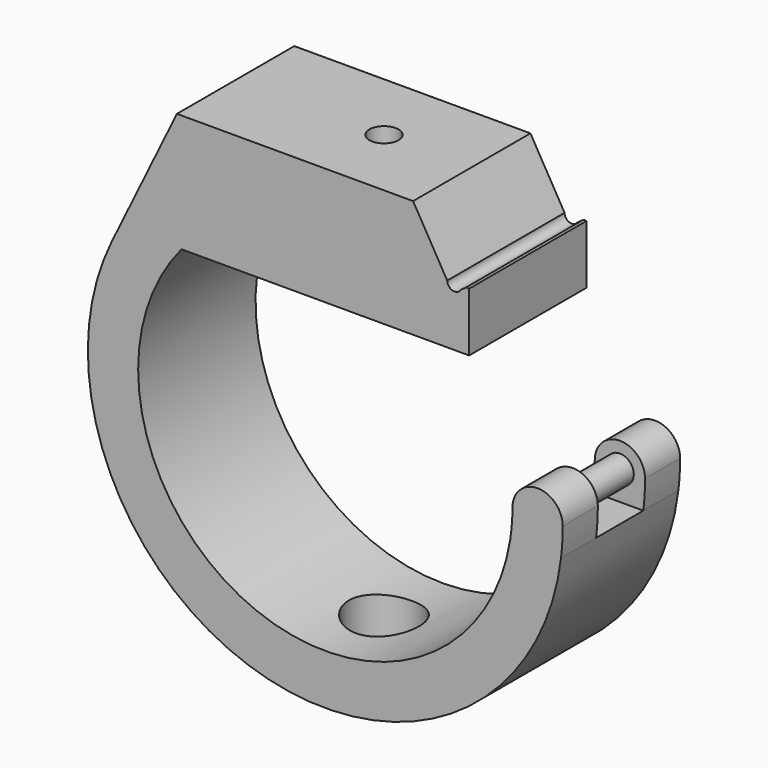
from build123d import *

# Parameters (mm, degrees)
F1_DEPTH  = 7.5
F2_DEPTH  = 17.6
F4_DEPTH  = 7.5
F6_DEPTH  = 25
F7_DEPTH  = 25.1
F8_R      = 2.5
F9_DEPTH  = 121.4
F10_DEPTH = 25.1
F11_R     = 6
F11_R_2   = 2.5
F12_DEPTH = 82
F14_DEPTH = 25.1


# Not quite as in the source:
# - a feature names something its author has since deleted; it is built from what else it names


with BuildPart() as f1:
    # F0 (on Front) → F1 (new body)
    with BuildSketch(Plane.XZ):
        with BuildLine():
            Line((24.609375, 40.625), (-25.390625, 40.625))
            Line((-25.390625, 40.625), (-25.390625, 31.7128804606))
            ThreePointArc((-25.390625, 31.7128804606), (-31.7255791152, 25.3747562511), (-36.5168539326, 17.8019662921))
            ThreePointArc((-36.5168539326, 17.8019662921), (-11.5217513517, -38.9568976022), (40.3254101185, -4.924624227))
            Line((40.3254101185, -4.924624227), (31.6393058234, -4.924624227))
            ThreePointArc((31.6393058234, -4.924624227), (-30.8610352871, -8.5378040369), (24.609375, 20.4860015345))
            Line((24.609375, 20.4860015345), (24.609375, 32.3228910698))
            Line((24.609375, 32.3228910698), (24.609375, 40.625))
        make_face()
        with BuildLine():
            Line((31.6393058234, -4.924624227), (40.3254101185, -4.924624227))
            ThreePointArc((40.3254101185, -4.924624227), (40.5500333604, -2.4668642988), (40.625, 0))
            ThreePointArc((40.625, 0), (36.3226342652, -4.3023657348), (32.0202685305, 0))
            ThreePointArc((32.0202685305, 0), (31.9248857895, -2.469668822), (31.6393058234, -4.924624227))
        make_face()
        with BuildLine():
            Line((38.6976342652, 0), (40.625, 0))
            ThreePointArc((40.625, 0), (36.3226342652, 4.3023657348), (32.0202685305, 0))
            Line((32.0202685305, 0), (33.9476342652, 0))
            ThreePointArc((33.9476342652, 0), (36.3226342652, 2.375), (38.6976342652, 0))
        make_face()
        with BuildLine():
            ThreePointArc((32.0202685305, 0), (36.3226342652, -4.3023657348), (40.625, 0))
            Line((40.625, 0), (38.6976342652, 0))
            ThreePointArc((38.6976342652, 0), (36.3226342652, -2.375), (33.9476342652, 0))
            Line((33.9476342652, 0), (32.0202685305, 0))
        make_face()
    extrude(amount=F1_DEPTH)

    # F0 (on Front) → F2 (join)
    with BuildSketch(Plane.XZ):
        with BuildLine():
            Line((24.609375, 40.625), (-25.390625, 40.625))
            Line((-25.390625, 40.625), (-25.390625, 31.7128804606))
            ThreePointArc((-25.390625, 31.7128804606), (-31.7255791152, 25.3747562511), (-36.5168539326, 17.8019662921))
            ThreePointArc((-36.5168539326, 17.8019662921), (-11.5217513517, -38.9568976022), (40.3254101185, -4.924624227))
            Line((40.3254101185, -4.924624227), (31.6393058234, -4.924624227))
            ThreePointArc((31.6393058234, -4.924624227), (-30.8610352871, -8.5378040369), (24.609375, 20.4860015345))
            Line((24.609375, 20.4860015345), (24.609375, 32.3228910698))
            Line((24.609375, 32.3228910698), (24.609375, 40.625))
        make_face()
    extrude(amount=F2_DEPTH)

    # F3 (on face) → F4 (join)
    with BuildSketch(Plane.XZ.offset(17.6)):
        with BuildLine():
            Line((24.609375, 40.625), (-25.390625, 40.625))
            Line((-25.390625, 40.625), (-25.390625, 31.7128804606))
            ThreePointArc((-25.390625, 31.7128804606), (-19.7822809369, -35.4831225505), (40.3254101185, -4.924624227))
            Line((40.3254101185, -4.924624227), (31.6393058234, -4.924624227))
            ThreePointArc((31.6393058234, -4.924624227), (-30.8610352871, -8.5378040369), (24.609375, 20.4860015345))
            Line((24.609375, 20.4860015345), (24.609375, 32.3228910698))
            Line((24.609375, 32.3228910698), (24.609375, 40.625))
        make_face()
        with BuildLine():
            Line((31.6393058234, -4.924624227), (40.3254101185, -4.924624227))
            ThreePointArc((40.3254101185, -4.924624227), (40.5500333604, -2.4668642988), (40.625, 0))
            ThreePointArc((40.625, 0), (36.3226342652, -4.3023657348), (32.0202685305, 0))
            ThreePointArc((32.0202685305, 0), (31.9248857895, -2.469668822), (31.6393058234, -4.924624227))
        make_face()
        with BuildLine():
            ThreePointArc((32.0202685305, 0), (36.3226342652, -4.3023657348), (40.625, 0))
            Line((40.625, 0), (38.6976342652, 0))
            ThreePointArc((38.6976342652, 0), (36.3226342652, -2.375), (33.9476342652, 0))
            Line((33.9476342652, 0), (32.0202685305, 0))
        make_face()
        with BuildLine():
            Line((38.6976342652, 0), (40.625, 0))
            ThreePointArc((40.625, 0), (36.3226342652, 4.3023657348), (32.0202685305, 0))
            Line((32.0202685305, 0), (33.9476342652, 0))
            ThreePointArc((33.9476342652, 0), (36.3226342652, 2.375), (38.6976342652, 0))
        make_face()
    extrude(amount=F4_DEPTH)

    # F5 (on face) → F6 (join)
    with BuildSketch(Plane.XZ.offset(25.1)):
        with BuildLine():
            Line((-24.609375, 20.4860015345), (24.609375, 20.4860015345))
            ThreePointArc((24.609375, 20.4860015345), (0, 32.0202685305), (-24.609375, 20.4860015345))
        make_face()
    extrude(amount=-F6_DEPTH)

    # F0 (on Front) → F7 (join)
    with BuildSketch(Plane.XZ):
        with BuildLine():
            Line((33.9476342652, 0), (38.6976342652, 0))
            ThreePointArc((38.6976342652, 0), (36.3226342652, 2.375), (33.9476342652, 0))
        make_face()
        with BuildLine():
            ThreePointArc((33.9476342652, 0), (36.3226342652, -2.375), (38.6976342652, 0))
            Line((38.6976342652, 0), (33.9476342652, 0))
        make_face()
    extrude(amount=F7_DEPTH)

    # F8 (on face) → F9 (cut)
    with BuildSketch(Plane.XY.offset(40.625)):
        with Locations((0, -12.55)):
            Circle(F8_R)
    extrude(amount=-F9_DEPTH, mode=Mode.SUBTRACT)

    # F0 (on Front) → F10 (join)
    with BuildSketch(Plane.XZ):
        with BuildLine():
            Line((-25.390625, 31.7128804606), (-25.390625, 40.625))
            Line((-25.390625, 40.625), (-36.5168539326, 17.8019662921))
            ThreePointArc((-36.5168539326, 17.8019662921), (-31.7255791152, 25.3747562511), (-25.390625, 31.7128804606))
        make_face()
    extrude(amount=F10_DEPTH)

    # F11 (on face) → F12 (cut)
    with BuildSketch(Plane(origin=(0, 0, 20.4860015345), x_dir=(1, 0, 0), z_dir=(0, 0, -1))):
        with Locations((0, 12.55)):
            Circle(F11_R)
        with Locations((0, 12.55)):
            Circle(F11_R_2, mode=Mode.SUBTRACT)
    extrude(amount=F12_DEPTH, mode=Mode.SUBTRACT)

    # F13 (on face) → F14 (cut)
    with BuildSketch(Plane.XZ.offset(25.1)):
        with BuildLine():
            ThreePointArc((23.1832968576, 29.9158197188), (23.3145518173, 30.2237646688), (23.359375, 30.5555007673))
            ThreePointArc((23.359375, 30.5555007673), (22.109375, 31.8055007673), (20.859375, 30.5555007673))
            ThreePointArc((20.859375, 30.5555007673), (21.7776389015, 29.35032395), (23.1832968576, 29.9158197188))
        make_face()
        with BuildLine():
            Line((24.085752666, 30.5555007673), (23.359375, 30.5555007673))
            ThreePointArc((23.359375, 30.5555007673), (23.3145518173, 30.2237646688), (23.1832968576, 29.9158197188))
            Line((23.1832968576, 29.9158197188), (24.085752666, 30.5555007673))
        make_face()
        with BuildLine():
            ThreePointArc((20.859375, 30.5555007673), (22.109375, 31.8055007673), (23.359375, 30.5555007673))
            Line((23.359375, 30.5555007673), (24.085752666, 30.5555007673))
            Line((24.085752666, 30.5555007673), (24.609375, 30.5555007673))
            Line((24.609375, 30.5555007673), (24.609375, 40.625))
            Line((24.609375, 40.625), (15.0185888633, 40.625))
            Line((15.0185888633, 40.625), (20.859375, 30.5555007673))
        make_face()
    extrude(amount=-F14_DEPTH, mode=Mode.SUBTRACT)


solid = f1.part
